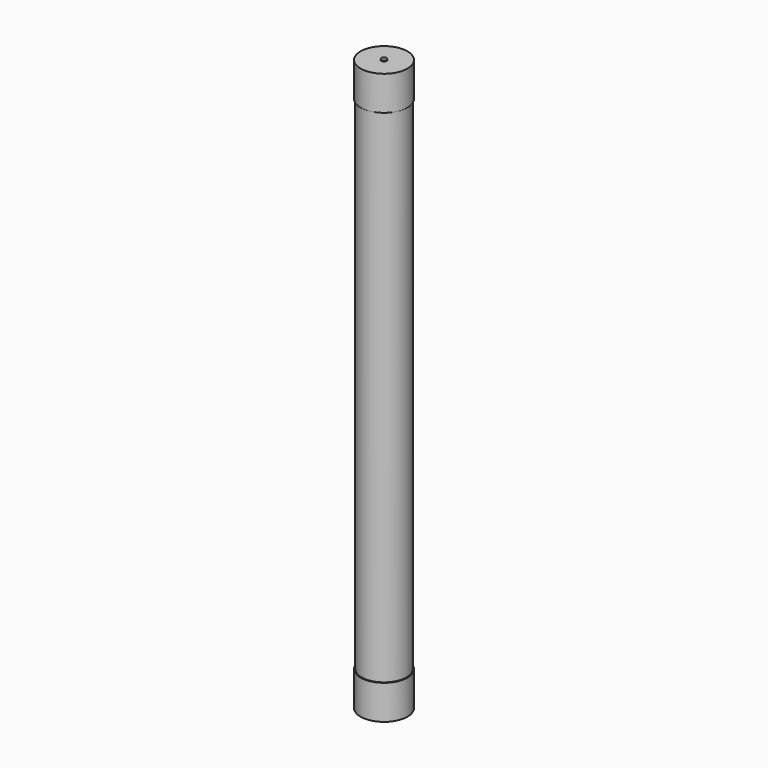
from build123d import *

# Parameters (mm, degrees)
F0_R     = 2.5
F1_DEPTH = 27.836615
F2_R     = 2.6
F2_R_2   = 2.5
F3_DEPTH = 3.813385
F4_R     = 2.6
F4_R_2   = 2.5
F5_DEPTH = 3.813385
F6_R     = 0.3
F7_DEPTH = 0.1
F8_R     = 0.3
F9_DEPTH = 0.1


with BuildPart() as f1:
    # F0 (on Top) → F1 (new body, symmetric)
    with BuildSketch(Plane.XY):
        Circle(F0_R)
    extrude(amount=F1_DEPTH, both=True)

    # F2 (on face) → F3 (join)
    with BuildSketch(Plane.XY.offset(27.836615)):
        Circle(F2_R)
        Circle(F2_R_2, mode=Mode.SUBTRACT)
        Circle(F2_R_2)
    extrude(amount=F3_DEPTH)

    # F4 (on face) → F5 (join)
    with BuildSketch(Plane(origin=(0, 0, -27.836615), x_dir=(1, 0, 0), z_dir=(0, 0, -1))):
        Circle(F4_R)
        Circle(F4_R_2, mode=Mode.SUBTRACT)
        Circle(F4_R_2)
    extrude(amount=F5_DEPTH)

    # F6 (on face) → F7 (join)
    with BuildSketch(Plane(origin=(0, 0, -31.65), x_dir=(1, 0, 0), z_dir=(0, 0, -1))):
        Circle(F6_R)
    extrude(amount=F7_DEPTH)

    # F8 (on face) → F9 (join)
    with BuildSketch(Plane.XY.offset(31.65)):
        Circle(F8_R)
    extrude(amount=F9_DEPTH)


solid = f1.part
